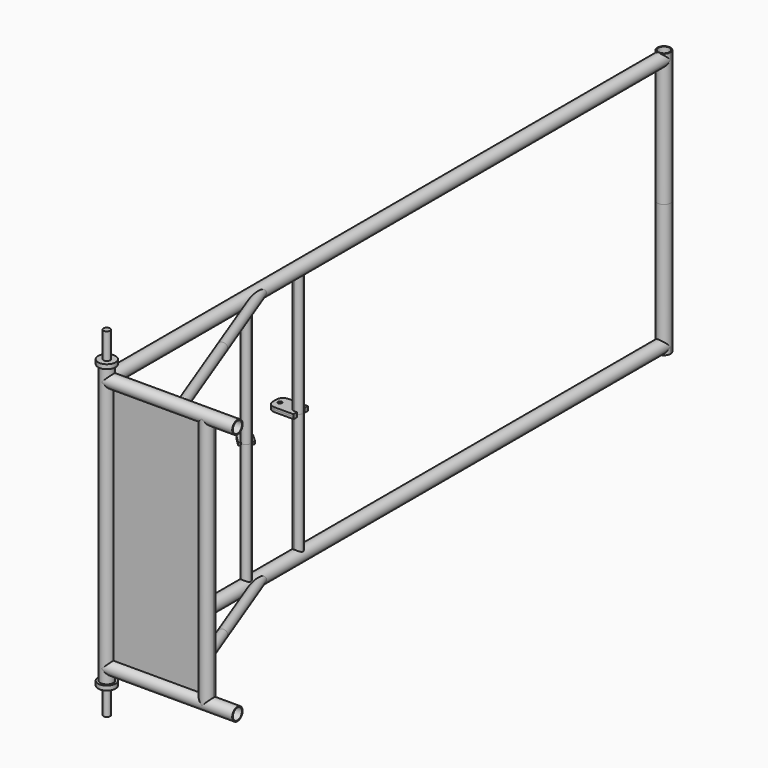
from build123d import *
from build123d import SkipClean  # not in build123d's __all__

# Parameters (mm, degrees)
F0_R           = 15
F0_R_2         = 13
F1_DEPTH       = 640
F2_R           = 20
F3_DEPTH       = 10
F4_R           = 7.5
F5_DEPTH       = 60
F6_R           = 20
F7_DEPTH       = 10
F8_R           = 7.5
F9_DEPTH       = 60
F11_R          = 15
F11_R_2        = 13
F12_DEPTH      = 300
F15_R          = 15
F15_R_2        = 13
F16_DEPTH      = 580
F18_DEPTH      = 1600
F22_R          = 15
F22_R_2        = 13
F23_DEPTH      = 305
F23_DEPTH_BACK = 305
F24_R          = 13
F25_DEPTH      = 700
F29_R          = 10.5
F29_R_2        = 8.5
F30_DEPTH      = 250
F30_DEPTH_BACK = 250
F32_R          = 8.5
F33_DEPTH      = 290
F33_DEPTH_BACK = 290
F32_R_2        = 4.5
F34_DEPTH      = 5
F34_DEPTH_BACK = 5
F32_R_3        = 3.25
F35_DEPTH      = 3
F35_DEPTH_BACK = 3
F37_W          = 230
F37_H          = 580
F38_DEPTH      = 2.5


with BuildPart() as f1:
    # F0 (on Top) → F1 (new body)
    with BuildSketch(Plane.XY):
        Circle(F0_R)
        Circle(F0_R_2, mode=Mode.SUBTRACT)
    extrude(amount=F1_DEPTH)

    # F2 (on face) → F3 (join)
    with BuildSketch(Plane.XY.offset(640)):
        Circle(F2_R)
    extrude(amount=F3_DEPTH)

    # F4 (on face) → F5 (join)
    with BuildSketch(Plane.XY.offset(650)):
        Circle(F4_R)
    extrude(amount=F5_DEPTH)

    # F6 (on face) → F7 (join)
    with BuildSketch(Plane(origin=(0, 0, 0), x_dir=(1, 0, 0), z_dir=(0, 0, -1))):
        Circle(F6_R)
    extrude(amount=F7_DEPTH)

    # F8 (on face) → F9 (join)
    with BuildSketch(Plane(origin=(0, 0, -10), x_dir=(1, 0, 0), z_dir=(0, 0, -1))):
        Circle(F8_R)
    extrude(amount=F9_DEPTH)

    # F11 (on offset) → F12 (join)
    with BuildSketch(Plane.YZ):
        with Locations((0, 30)):
            Circle(F11_R)
        with Locations((0, 30)):
            Circle(F11_R_2, mode=Mode.SUBTRACT)
        with Locations((0, 610)):
            Circle(F11_R)
        with Locations((0, 610)):
            Circle(F11_R_2, mode=Mode.SUBTRACT)
    extrude(amount=F12_DEPTH)

    # F15 (on offset) → F16 (join)
    with BuildSketch(Plane.XY.offset(30)):
        with Locations((230, 0)):
            Circle(F15_R)
        with Locations((230, 0)):
            Circle(F15_R_2, mode=Mode.SUBTRACT)
    extrude(amount=F16_DEPTH)

    # F17 (on Front) → F18 (join)
    with BuildSketch(Plane.XZ):
        with BuildLine():
            ThreePointArc((0, 15), (10.6066017178, 19.3933982822), (15, 30))
            ThreePointArc((15, 30), (10.6066017178, 40.6066017178), (0, 45))
            Line((0, 45), (0, 43))
            ThreePointArc((0, 43), (9.1923881554, 39.1923881554), (13, 30))
            ThreePointArc((13, 30), (9.1923881554, 20.8076118446), (0, 17))
            Line((0, 17), (0, 15))
        make_face()
        with BuildLine():
            ThreePointArc((15, 610), (-10.6066017178, 620.6066017178), (0, 595))
            ThreePointArc((0, 595), (10.6066017178, 599.3933982822), (15, 610))
        make_face()
        with BuildLine():
            ThreePointArc((13, 610), (9.1923881554, 600.8076118446), (0, 597))
            ThreePointArc((0, 597), (-9.1923881554, 619.1923881554), (13, 610))
        make_face(mode=Mode.SUBTRACT)
        with BuildLine():
            Line((0, 43), (0, 45))
            ThreePointArc((0, 45), (-15, 30), (0, 15))
            Line((0, 15), (0, 17))
            ThreePointArc((0, 17), (-13, 30), (0, 43))
        make_face()
    extrude(amount=-F18_DEPTH)

    # F22 (on line) → F23 (join, two sides)
    with BuildSketch(Plane.XY.offset(320)) as f23_sk:
        with Locations((0, 1600)):
            Circle(F22_R)
        with Locations((0, 1600)):
            Circle(F22_R_2, mode=Mode.SUBTRACT)
    extrude(amount=F23_DEPTH)
    extrude(f23_sk.sketch, amount=-F23_DEPTH_BACK)

    # F24 (on face) → F25 (cut)
    with BuildSketch(Plane(origin=(0, 0, 15), x_dir=(1, 0, 0), z_dir=(0, 0, -1))):
        with Locations((0, -1600)):
            Circle(F24_R)
    extrude(amount=-F25_DEPTH, mode=Mode.SUBTRACT)

    # F29 (on line) → F30 (join, two sides)
    with BuildSketch(Plane(origin=(-63.768366465, 168.7986171132, 0), x_dir=(-0.9354720937, -0.3534005687, 0), z_dir=(-0.3534005687, 0.9354720937, 0))) as f30_sk:
        with Locations((-159.0302559234, 30)):
            Circle(F29_R)
        with Locations((-159.0302559234, 30)):
            Circle(F29_R_2, mode=Mode.SUBTRACT)
        with Locations((-159.0302559234, 610)):
            Circle(F29_R)
        with Locations((-159.0302559234, 610)):
            Circle(F29_R_2, mode=Mode.SUBTRACT)
    extrude(amount=F30_DEPTH)
    extrude(f30_sk.sketch, amount=-F30_DEPTH_BACK)

    # F32 (on line) → F33 (join, two sides)
    with BuildSketch(Plane(origin=(0, 0, 320), x_dir=(1, 0, 0), z_dir=(0, 0, -1))) as f33_sk:
        with BuildLine():
            ThreePointArc((0, -560.5), (7.4246212025, -557.4246212025), (10.5, -550))
            ThreePointArc((10.5, -550), (7.4246212025, -542.5753787975), (0, -539.5))
            ThreePointArc((0, -539.5), (-7.4246212025, -542.5753787975), (-10.5, -550))
            ThreePointArc((-10.5, -550), (-7.4246212025, -557.4246212025), (0, -560.5))
        make_face()
        with Locations((0, -550)):
            Circle(F32_R, mode=Mode.SUBTRACT)
        with BuildLine():
            ThreePointArc((7.1609827807, -407.679213867), (9.629130781, -404.1868652237), (10.5, -400))
            ThreePointArc((10.5, -400), (4.1868652237, -390.370869219), (-7.1609827807, -392.320786133))
            ThreePointArc((-7.1609827807, -392.320786133), (-10.4936036837, -399.6335552846), (-7.679213867, -407.1609827807))
            ThreePointArc((-7.679213867, -407.1609827807), (-0.3664447154, -410.4936036837), (7.1609827807, -407.679213867))
        make_face()
        with Locations((0, -400)):
            Circle(F32_R, mode=Mode.SUBTRACT)
    extrude(amount=F33_DEPTH)
    extrude(f33_sk.sketch, amount=-F33_DEPTH_BACK)

    # F32 (on line) → F34 (join, two sides)
    with BuildSketch(Plane(origin=(0, 0, 320), x_dir=(1, 0, 0), z_dir=(0, 0, -1))) as f34_sk:
        with BuildLine():
            ThreePointArc((-10.5, -550), (-7.4246212025, -542.5753787975), (0, -539.5))
            Line((0, -539.5), (5.5, -539.5))
            Line((5.5, -539.5), (5.5, -529.5))
            Line((5.5, -529.5), (-39.5, -529.5))
            ThreePointArc((-39.5, -529.5), (-50.1066017178, -533.8933982822), (-54.5, -544.5))
            Line((-54.5, -544.5), (-54.5, -555.5))
            ThreePointArc((-54.5, -555.5), (-50.1066017178, -566.1066017178), (-39.5, -570.5))
            Line((-39.5, -570.5), (5.5, -570.5))
            Line((5.5, -570.5), (5.5, -560.5))
            Line((5.5, -560.5), (0, -560.5))
            ThreePointArc((0, -560.5), (-7.4246212025, -557.4246212025), (-10.5, -550))
        make_face()
        with Locations((-42.5, -550)):
            Circle(F32_R_2, mode=Mode.SUBTRACT)
    extrude(amount=F34_DEPTH)
    extrude(f34_sk.sketch, amount=-F34_DEPTH_BACK)

    # F32 (on line) → F35 (join, two sides)
    with BuildSketch(Plane(origin=(0, 0, 320), x_dir=(1, 0, 0), z_dir=(0, 0, -1))) as f35_sk:
        with BuildLine():
            ThreePointArc((-7.679213867, -407.1609827807), (-10.4936036837, -399.6335552846), (-7.1609827807, -392.320786133))
            Line((-7.1609827807, -392.320786133), (-3.1385374218, -388.5697951527))
            Line((-3.1385374218, -388.5697951527), (-6.5023567325, -384.9625405776))
            Line((-6.5023567325, -384.9625405776), (-24.1783092962, -402.6384931412))
            ThreePointArc((-24.1783092962, -402.6384931412), (-27.1072414843, -409.7095609531), (-24.1783092962, -416.780628765))
            Line((-24.1783092962, -416.780628765), (-17.0562428513, -423.9026952099))
            ThreePointArc((-17.0562428513, -423.9026952099), (-10.1596991038, -426.8301043496), (-3.1651914388, -424.1451644142))
            Line((-3.1651914388, -424.1451644142), (14.5934199399, -407.5849913948))
            Line((14.5934199399, -407.5849913948), (11.1834281396, -403.9282228867))
            Line((11.1834281396, -403.9282228867), (7.1609827807, -407.679213867))
            ThreePointArc((7.1609827807, -407.679213867), (-0.3664447154, -410.4936036837), (-7.679213867, -407.1609827807))
        make_face()
        with Locations((-15.0817303242, -414.5634992379)):
            Circle(F32_R_3, mode=Mode.SUBTRACT)
    extrude(amount=F35_DEPTH)
    extrude(f35_sk.sketch, amount=-F35_DEPTH_BACK)

    # F37 (on face) → F38 (join)
    with BuildSketch(Plane(origin=(0, 0, 0), x_dir=(-1, 0, 0), z_dir=(0, 1, 0))):
        with Locations((-115, 320)):
            Rectangle(F37_W, F37_H)
    with SkipClean():  # cleaning this boolean's faces spoils the solid; the shape is the same uncleaned
        extrude(amount=F38_DEPTH)


solid = f1.part
